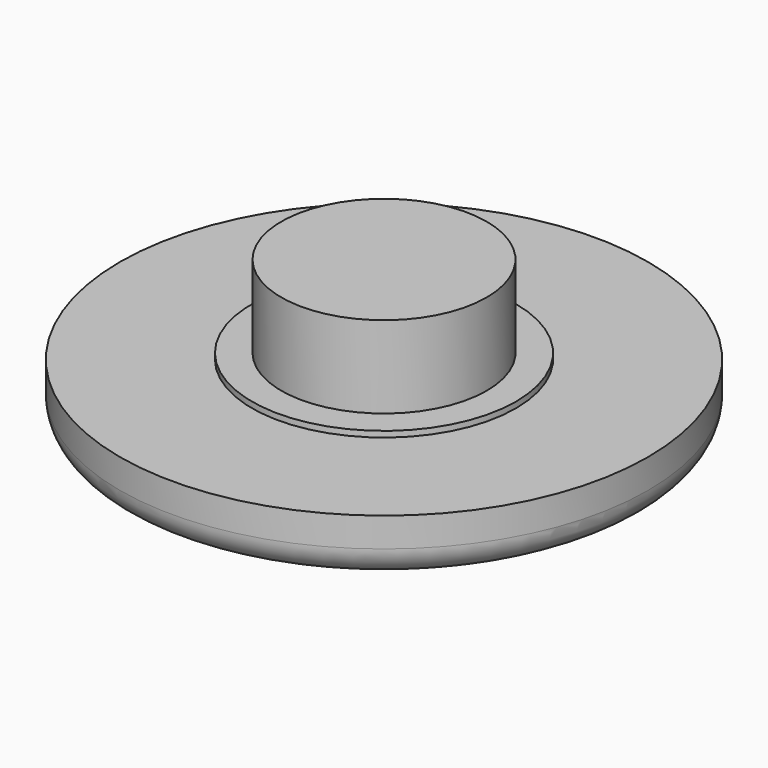
from build123d import *

# Parameters (mm, degrees)
F0_R         = 9
F1_DEPTH     = 2
F2_R         = 3.5
F3_DEPTH     = 3
F4_R         = 1
F5_TEXT_SIZE = 16.6666666667
F6_DEPTH     = 1.5
F7_R         = 4.5
F7_R_2       = 3.5
F8_DEPTH     = 0.2


# Not quite as in the source:
# - Text() gives the source's letters only with a copy of the font that has no kerning and outlines rounded to 1/6400 em; it was checked with that copy


with BuildPart() as f1:
    # F0 (on Top) → F1 (new body)
    with BuildSketch(Plane.XY):
        Circle(F0_R)
    extrude(amount=F1_DEPTH)

    # F2 (on face) → F3 (join)
    with BuildSketch(Plane.XY.offset(2)):
        Circle(F2_R)
    extrude(amount=F3_DEPTH)

    # F4
    f4_edges = [f1.edges().sort_by_distance(p)[0] for p in [
        (-9, 0, 0),
    ]]
    fillet(f4_edges, radius=F4_R)

    # F5 (on face) → F6 (cut)
    with BuildSketch(Plane(origin=(0, 0, 0), x_dir=(1, 0, 0), z_dir=(0, 0, -1))):
        with Locations((-6.5677284001, -5.9009650626)):
            Text('O', F5_TEXT_SIZE, font='Open Sans', font_style=FontStyle.BOLD, text_align=(TextAlign.LEFT, TextAlign.BOTTOM))
    extrude(amount=-F6_DEPTH, mode=Mode.SUBTRACT)

    # F7 (on face) → F8 (join)
    with BuildSketch(Plane.XY.offset(2)):
        Circle(F7_R)
        Circle(F7_R_2, mode=Mode.SUBTRACT)
    extrude(amount=F8_DEPTH)


solid = f1.part
